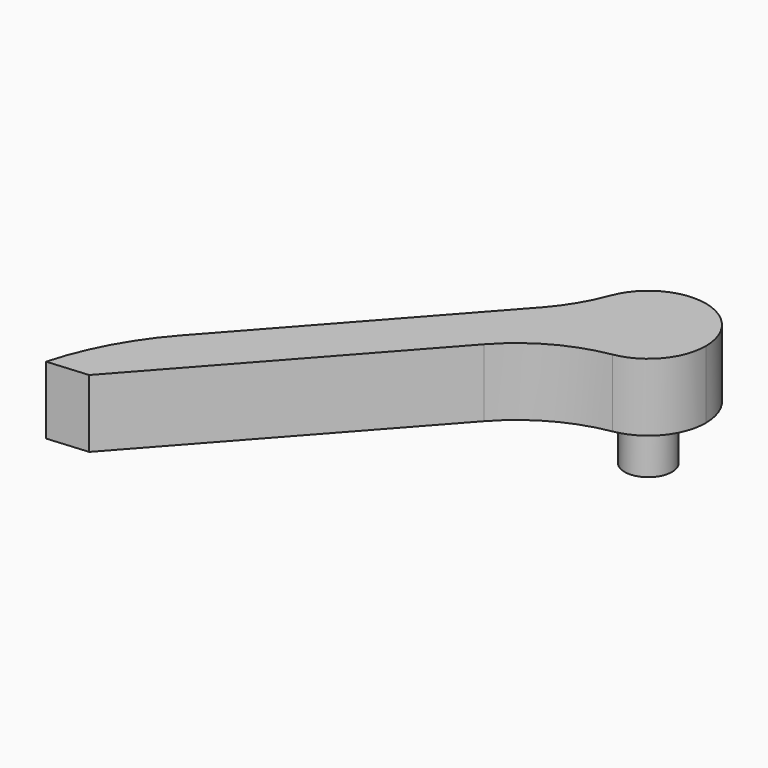
from build123d import *

# Parameters (mm, degrees)
F0_R          = 1.75
F1_DEPTH      = 5
F2_DEPTH      = 4
F2_DEPTH_BACK = 5
F3_T1_DEPTH   = 35.3628033386
F4_R          = 11.3728971787


# Not quite as in the source:
# - a fillet or chamfer that OpenCascade refuses, or shapes differently, is made with other operations: its cross-section is extruded or revolved along the edge and cut away or added


with BuildPart() as f1:
    # F0 (on Top) → F1 (new body)
    with BuildSketch(Plane.XY):
        with BuildLine():
            ThreePointArc((-2.5631937321, 5.253964594), (1.7029722297, 5.2256762725), (3.8442630819, 8.9156418184))
            ThreePointArc((3.8442630819, 8.9156418184), (-0.4057369181, 13.1656418184), (-4.6557369181, 8.9156418184))
            ThreePointArc((-4.6557369181, 8.9156418184), (-4.095702464, 6.8069326705), (-2.5631937321, 5.253964594))
        make_face()
        with Locations((-0.4057369181, 8.9156418184)):
            Circle(F0_R, mode=Mode.SUBTRACT)
        with BuildLine():
            ThreePointArc((-2.5631937321, 5.253964594), (-4.095702464, 6.8069326705), (-4.6557369181, 8.9156418184))
            Line((-4.6557369181, 8.9156418184), (-24.6422081436, -13.4571310977))
            Line((-24.6422081436, -13.4571310977), (-21.6591717548, -16.1219939277))
            Line((-21.6591717548, -16.1219939277), (-2.5631937321, 5.253964594))
        make_face()
        Polygon((-21.6591717548, -16.1219939277), (-24.6422081436, -13.4571310977), (-24.6422081436, -16.1219939277), (-24.6422081436, -16.3715779781), align=None)
    extrude(amount=F1_DEPTH)

    # F0 (on Top) → F2 (join, two sides)
    with BuildSketch(Plane.XY) as f2_sk:
        with Locations((-0.4057369181, 8.9156418184)):
            Circle(F0_R)
    extrude(amount=-F2_DEPTH)
    extrude(f2_sk.sketch, amount=F2_DEPTH_BACK)

    # F3: fillet of radius 18.4809579153 on 1 edges, made by hand

    # F3_s2 → F3_t1 (cut)
    with BuildSketch(Plane.XY.offset(-15.1814016693)):
        with BuildLine():
            ThreePointArc((-20.5965728419, -8.9284637364), (-23.0516277567, -12.4150823252), (-24.6422081436, -16.3715779781))
            Line((-24.6422081436, -16.3715779781), (-24.6422081436, -13.4571310977))
            Line((-24.6422081436, -13.4571310977), (-20.5965728419, -8.9284637364))
        make_face()
    extrude(amount=F3_T1_DEPTH, mode=Mode.SUBTRACT)

    # F4
    f4_edges = [f1.edges().sort_by_distance(p)[0] for p in [
        (-2.563194, 5.253965, 2.5),
        (-4.655737, 8.915642, 2.5),
    ]]
    fillet(f4_edges, radius=F4_R)


solid = f1.part
